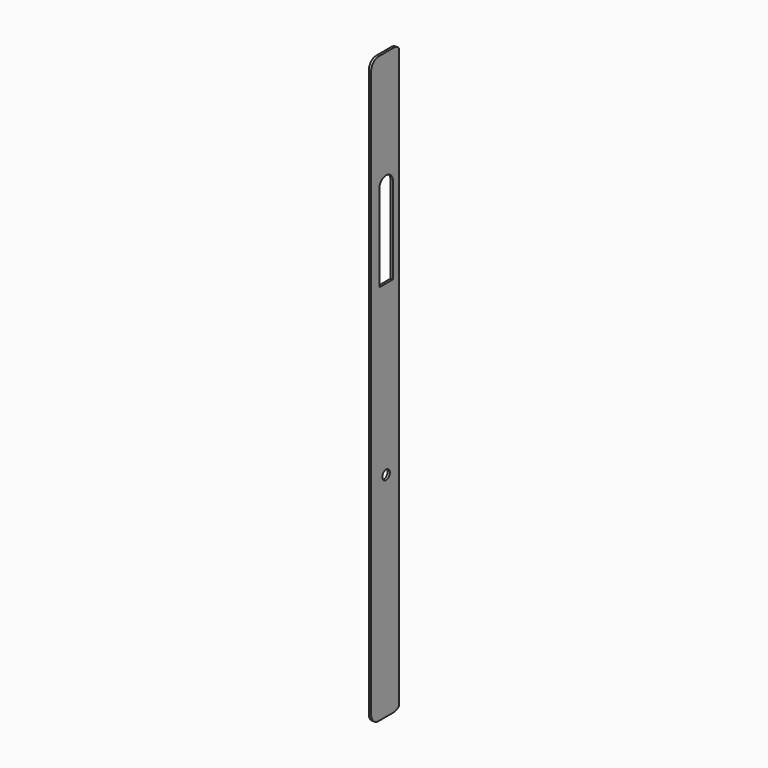
from build123d import *

# Parameters (mm, degrees)
F0_W        = 8
F0_H        = 125
F1_DEPTH    = 0.5
F2_R        = 2
F3_R        = 1
F4_DEPTH    = 12.5
F5_T1_DEPTH = 125.3718610795


# Not quite as in the source:
# - a fillet or chamfer that OpenCascade refuses, or shapes differently, is made with other operations: its cross-section is extruded or revolved along the edge and cut away or added


with BuildPart() as f1:
    # F0 (on Right) → F1 (new body)
    with BuildSketch(Plane.YZ):
        with Locations((30.2877472714, 96.0264432559)):
            Rectangle(F0_W, F0_H)
    extrude(amount=F1_DEPTH)

    # F2
    f2_edges = [f1.edges().sort_by_distance(p)[0] for p in [
        (0.25, 26.287747, 158.526443),
        (0.25, 34.287747, 158.526443),
        (0.25, 34.287747, 33.526443),
        (0.25, 26.287747, 33.526443),
    ]]
    fillet(f2_edges, radius=F2_R)

    # F3 (on face) → F4 (cut, symmetric)
    with BuildSketch(Plane.YZ.offset(0.5)):
        with BuildLine():
            Line((28.4577472714, 133.5264432559), (28.4577472714, 115.0264432559))
            Line((28.4577472714, 115.0264432559), (32.1177472714, 115.0264432559))
            Line((32.1177472714, 115.0264432559), (32.1177472714, 133.5264432559))
            ThreePointArc((32.1177472714, 133.5264432559), (30.2877472714, 135.3564432559), (28.4577472714, 133.5264432559))
        make_face()
        with Locations((30.2877472714, 79.0264432559)):
            Circle(F3_R)
    extrude(amount=F4_DEPTH, both=True, mode=Mode.SUBTRACT)

    # F5: chamfer of 0.5 on 1 edges, made by hand

    # F5_s2 → F5_t1 (cut)
    with BuildSketch(Plane.XY.offset(33.3405127162)):
        Polygon((0.5, 33.7877472714), (0, 34.2877472714), (0.5, 34.2877472714), align=None)
    extrude(amount=F5_T1_DEPTH, mode=Mode.SUBTRACT)


solid = f1.part
